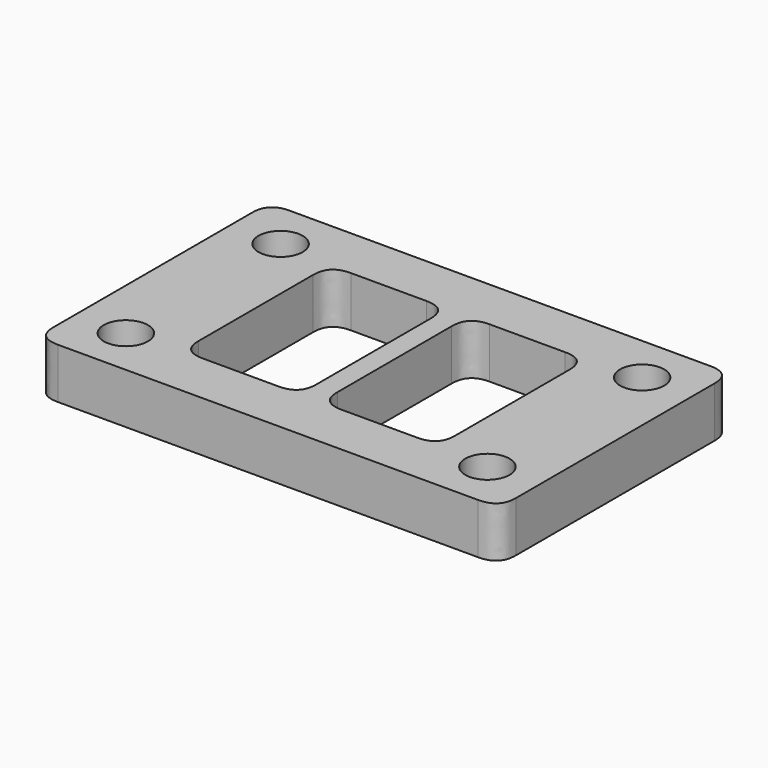
from build123d import *

# Parameters (mm, degrees)
F0_W        = 110
F0_H        = 69
F0_R        = 5.25
F0_W_2      = 5
F0_H_2      = 44
F1_DEPTH    = 12
F2_T1_DEPTH = 12
F2_T3_DEPTH = 37


# Not quite as in the source:
# - a fillet or chamfer that OpenCascade refuses, or shapes differently, is made with other operations: its cross-section is extruded or revolved along the edge and cut away or added


with BuildPart() as f1:
    # F0 (on Top) → F1 (new body)
    with BuildSketch(Plane.XY):
        Rectangle(F0_W, F0_H)
        with Locations((-43, -23)):
            Circle(F0_R, mode=Mode.SUBTRACT)
        with Locations((43, -23)):
            Circle(F0_R, mode=Mode.SUBTRACT)
        with Locations((-43, 23)):
            Circle(F0_R, mode=Mode.SUBTRACT)
        Polygon((30.5, 22), (30.5, -22), (2.5, -22), (-2.5, -22), (-30.5, -22), (-30.5, 22), (-2.5, 22), (2.5, 22), align=None, mode=Mode.SUBTRACT)
        with Locations((43, 23)):
            Circle(F0_R, mode=Mode.SUBTRACT)
        Rectangle(F0_W_2, F0_H_2)
    extrude(amount=F1_DEPTH)

    # F2: fillet of radius 5 on 12 edges, made by hand

    # F2_s2 → F2_t1 (join)
    with BuildSketch(Plane.XY):
        with BuildLine():
            add(Edge.make_bspline(
                [(-30.5, 17), (-30.5, 22), (-25.5, 22)],
                knots=[0, 0, 0, 1, 1, 1], degree=2, weights=[1, 1, 1]))
            Line((-25.5, 22), (-30.5, 22))
            Line((-30.5, 22), (-30.5, 17))
        make_face()
        with BuildLine():
            add(Edge.make_bspline(
                [(2.5, 17), (2.5, 22), (7.5, 22)],
                knots=[0, 0, 0, 1, 1, 1], degree=2, weights=[1, 1, 1]))
            Line((7.5, 22), (2.5, 22))
            Line((2.5, 22), (2.5, 17))
        make_face()
        with BuildLine():
            add(Edge.make_bspline(
                [(30.5, -17), (30.5, -22), (25.5, -22)],
                knots=[0, 0, 0, 1, 1, 1], degree=2, weights=[1, 1, 1]))
            Line((25.5, -22), (30.5, -22))
            Line((30.5, -22), (30.5, -17))
        make_face()
        with BuildLine():
            add(Edge.make_bspline(
                [(-7.5, -22), (-2.5, -22), (-2.5, -17)],
                knots=[0, 0, 0, 1, 1, 1], degree=2, weights=[1, 1, 1]))
            Line((-2.5, -17), (-2.5, -22))
            Line((-2.5, -22), (-7.5, -22))
        make_face()
        with BuildLine():
            add(Edge.make_bspline(
                [(30.5, 17), (30.5, 22), (25.5, 22)],
                knots=[0, 0, 0, 1, 1, 1], degree=2, weights=[1, 1, 1]))
            Line((25.5, 22), (30.5, 22))
            Line((30.5, 22), (30.5, 17))
        make_face()
        with BuildLine():
            add(Edge.make_bspline(
                [(-7.5, 22), (-2.5, 22), (-2.5, 17)],
                knots=[0, 0, 0, 1, 1, 1], degree=2, weights=[1, 1, 1]))
            Line((-2.5, 17), (-2.5, 22))
            Line((-2.5, 22), (-7.5, 22))
        make_face()
        with BuildLine():
            add(Edge.make_bspline(
                [(-25.5, -22), (-30.5, -22), (-30.5, -17)],
                knots=[0, 0, 0, 1, 1, 1], degree=2, weights=[1, 1, 1]))
            Line((-30.5, -17), (-30.5, -22))
            Line((-30.5, -22), (-25.5, -22))
        make_face()
        with BuildLine():
            add(Edge.make_bspline(
                [(7.5, -22), (2.5, -22), (2.5, -17)],
                knots=[0, 0, 0, 1, 1, 1], degree=2, weights=[1, 1, 1]))
            Line((2.5, -17), (2.5, -22))
            Line((2.5, -22), (7.5, -22))
        make_face()
    extrude(amount=F2_T1_DEPTH)

    # F2_s4 → F2_t3 (cut)
    with BuildSketch(Plane.XY.offset(-12.5)):
        with BuildLine():
            add(Edge.make_bspline(
                [(55, -29.5), (55, -34.5), (50, -34.5)],
                knots=[0, 0, 0, 1, 1, 1], degree=2, weights=[1, 1, 1]))
            Line((50, -34.5), (55, -34.5))
            Line((55, -34.5), (55, -29.5))
        make_face()
        with BuildLine():
            add(Edge.make_bspline(
                [(50, 34.5), (55, 34.5), (55, 29.5)],
                knots=[0, 0, 0, 1, 1, 1], degree=2, weights=[1, 1, 1]))
            Line((55, 29.5), (55, 34.5))
            Line((55, 34.5), (50, 34.5))
        make_face()
        with BuildLine():
            add(Edge.make_bspline(
                [(-55, -29.5), (-55, -34.5), (-50, -34.5)],
                knots=[0, 0, 0, 1, 1, 1], degree=2, weights=[1, 1, 1]))
            Line((-50, -34.5), (-55, -34.5))
            Line((-55, -34.5), (-55, -29.5))
        make_face()
        with BuildLine():
            add(Edge.make_bspline(
                [(-50, 34.5), (-55, 34.5), (-55, 29.5)],
                knots=[0, 0, 0, 1, 1, 1], degree=2, weights=[1, 1, 1]))
            Line((-55, 29.5), (-55, 34.5))
            Line((-55, 34.5), (-50, 34.5))
        make_face()
    extrude(amount=F2_T3_DEPTH, mode=Mode.SUBTRACT)


solid = f1.part
